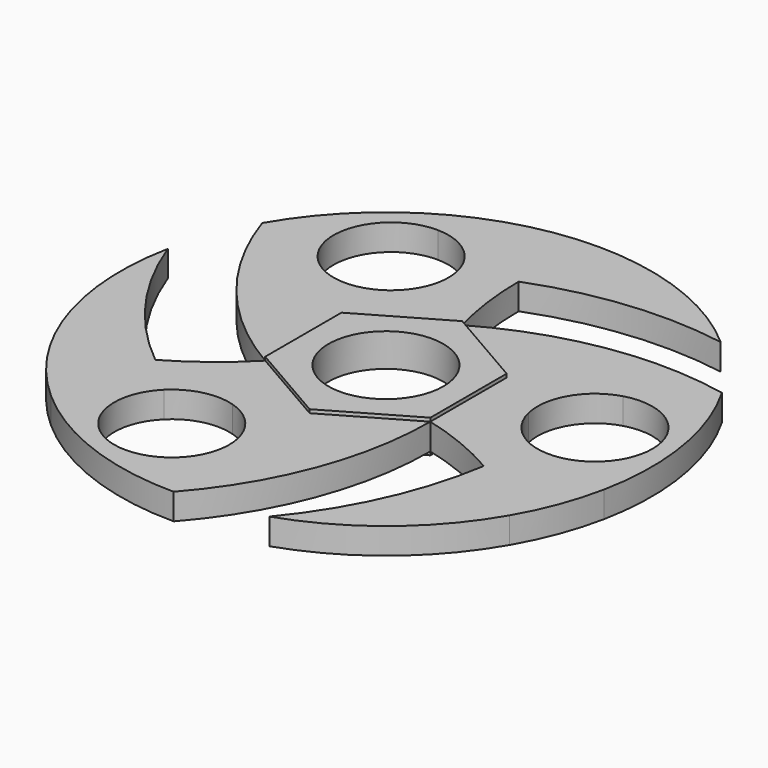
from build123d import *

# Parameters (mm, degrees)
F0_R     = 11
F1_DEPTH = 2.5
F2_DEPTH = 3.175


with BuildPart() as f1:
    # F0 (on Top) → F1 (new body, symmetric)
    with BuildSketch(Plane.XY):
        with BuildLine():
            ThreePointArc((20.292549, -3.190621), (15.603867, 0.493492), (10.5871, 3.716606))
            Line((10.5871, 3.716606), (10.5871, -14.535403))
            ThreePointArc((10.5871, -14.535403), (18.397515, -17.131664), (25.787001, -20.756393))
            ThreePointArc((25.787001, -20.756393), (32.620851, -25.343511), (38.774487, -30.809399))
            ThreePointArc((38.774487, -30.809399), (34.310981, -20.571216), (28.105483, -11.284932))
            ThreePointArc((28.105483, -11.284932), (23.085978, -8.312122), (20.292549, -3.190621))
        make_face()
        Polygon((10.5871, -14.535403), (10.5871, 3.716606), (-5.219603, 12.84261), (-21.026306, 3.716606), (-21.026306, -14.535403), (-5.219603, -23.661407), align=None)
        with Locations((-5.219603, -5.409399)):
            Circle(F0_R, mode=Mode.SUBTRACT)
        with BuildLine():
            Line((-5.219603, 12.84261), (10.5871, 3.716606))
            ThreePointArc((10.5871, 3.716606), (16.740736, 9.182493), (23.574586, 13.769612))
            ThreePointArc((23.574586, 13.769612), (30.964072, 17.39434), (38.774487, 19.990601))
            ThreePointArc((38.774487, 19.990601), (16.122412, 20.448153), (-5.219603, 12.84261))
        make_face()
        with BuildLine():
            ThreePointArc((-5.219603, -56.209399), (6.502686, -36.820901), (10.5871, -14.535403))
            Line((10.5871, -14.535403), (-5.219603, -23.661407))
            ThreePointArc((-5.219603, -23.661407), (-3.562824, -31.723556), (-3.007188, -39.935403))
            ThreePointArc((-3.007188, -39.935403), (-3.562824, -48.14725), (-5.219603, -56.209399))
        make_face()
        with BuildLine():
            Line((-21.026306, 3.716606), (-5.219603, 12.84261))
            ThreePointArc((-5.219603, 12.84261), (-6.876383, 20.904759), (-7.432019, 29.116606))
            ThreePointArc((-7.432019, 29.116606), (-6.876383, 37.328452), (-5.219603, 45.390601))
            ThreePointArc((-5.219603, 45.390601), (-11.854376, 36.406), (-16.793785, 26.388739))
            ThreePointArc((-16.793785, 26.388739), (-16.522621, 25.000927), (-16.431732, 23.589795))
            ThreePointArc((-16.431732, 23.589795), (-17.335201, 19.224012), (-19.897197, 15.575384))
            ThreePointArc((-19.897197, 15.575384), (-20.743392, 9.672811), (-21.026306, 3.716606))
        make_face()
        with BuildLine():
            ThreePointArc((38.774487, 19.990601), (30.964072, 17.39434), (23.574586, 13.769612))
            ThreePointArc((23.574586, 13.769612), (25.809021, 11.881337), (27.960245, 9.898783))
            ThreePointArc((27.960245, 9.898783), (37.61704, 8.114843), (42.0005, -0.672728))
            ThreePointArc((42.0005, -0.672728), (41.596743, -3.625628), (40.415115, -6.361755))
            ThreePointArc((40.415115, -6.361755), (42.663166, -10.833694), (44.576485, -15.458754))
            ThreePointArc((44.576485, -15.458754), (44.913356, 2.795866), (38.774487, 19.990601))
        make_face()
        with BuildLine():
            ThreePointArc((-16.054161, -28.612959), (-10.519285, -26.394499), (-5.219603, -23.661407))
            Line((-5.219603, -23.661407), (-21.026306, -14.535403))
            ThreePointArc((-21.026306, -14.535403), (-27.179942, -20.00129), (-34.013792, -24.588409))
            ThreePointArc((-34.013792, -24.588409), (-41.403278, -28.213137), (-49.213694, -30.809399))
            ThreePointArc((-49.213694, -30.809399), (-38.115414, -32.06298), (-26.970508, -31.332003))
            ThreePointArc((-26.970508, -31.332003), (-21.886226, -28.471389), (-16.054161, -28.612959))
        make_face()
        with BuildLine():
            ThreePointArc((38.774487, -30.809399), (32.620851, -25.343511), (25.787001, -20.756393))
            ThreePointArc((25.787001, -20.756393), (20.588854, -38.154406), (10.975444, -53.558754))
            ThreePointArc((10.975444, -53.558754), (26.952844, -44.723183), (38.774487, -30.809399))
        make_face()
        with BuildLine():
            ThreePointArc((-38.820645, -43.509399), (-23.180116, -52.928448), (-5.219603, -56.209399))
            ThreePointArc((-5.219603, -56.209399), (-3.562824, -48.14725), (-3.007188, -39.935403))
            ThreePointArc((-3.007188, -39.935403), (-5.759699, -40.926344), (-8.552253, -41.798082))
            ThreePointArc((-8.552253, -41.798082), (-17.801202, -50.052392), (-28.861727, -44.454046))
            ThreePointArc((-28.861727, -44.454046), (-33.858565, -44.164946), (-38.820645, -43.509399))
        make_face()
        with BuildLine():
            Line((-21.026306, -14.535403), (-21.026306, 3.716606))
            ThreePointArc((-21.026306, 3.716606), (-28.836722, 6.312867), (-36.226208, 9.937595))
            ThreePointArc((-36.226208, 9.937595), (-43.060058, 14.524714), (-49.213694, 19.990601))
            ThreePointArc((-49.213694, 19.990601), (-38.283907, 0.144553), (-21.026306, -14.535403))
        make_face()
        with BuildLine():
            ThreePointArc((-5.219603, 45.390601), (-6.876383, 37.328452), (-7.432019, 29.116606))
            ThreePointArc((-7.432019, 29.116606), (10.234176, 33.313884), (28.381438, 32.690601))
            ThreePointArc((28.381438, 32.690601), (12.740909, 42.10965), (-5.219603, 45.390601))
        make_face()
        with BuildLine():
            ThreePointArc((40.415115, -6.361755), (35.085314, -10.886165), (28.105483, -11.284932))
            ThreePointArc((28.105483, -11.284932), (34.310981, -20.571216), (38.774487, -30.809399))
            ThreePointArc((38.774487, -30.809399), (42.299445, -23.369911), (44.576485, -15.458754))
            ThreePointArc((44.576485, -15.458754), (42.663166, -10.833694), (40.415115, -6.361755))
        make_face()
        with BuildLine():
            ThreePointArc((-49.213694, -30.809399), (-44.533388, -37.581846), (-38.820645, -43.509399))
            ThreePointArc((-38.820645, -43.509399), (-33.858565, -44.164946), (-28.861727, -44.454046))
            ThreePointArc((-28.861727, -44.454046), (-30.115081, -37.576098), (-26.970508, -31.332003))
            ThreePointArc((-26.970508, -31.332003), (-38.115414, -32.06298), (-49.213694, -30.809399))
        make_face()
        with BuildLine():
            ThreePointArc((-49.213694, 19.990601), (-43.060058, 14.524714), (-36.226208, 9.937595))
            ThreePointArc((-36.226208, 9.937595), (-35.708132, 12.816811), (-35.066802, 15.671102))
            ThreePointArc((-35.066802, 15.671102), (-37.59077, 27.808082), (-27.212198, 34.587604))
            ThreePointArc((-27.212198, 34.587604), (-24.463411, 38.770444), (-21.41465, 42.739957))
            ThreePointArc((-21.41465, 42.739957), (-37.392051, 33.904386), (-49.213694, 19.990601))
        make_face()
        with BuildLine():
            ThreePointArc((-16.793785, 26.388739), (-11.854376, 36.406), (-5.219603, 45.390601))
            ThreePointArc((-5.219603, 45.390601), (-13.424868, 44.723561), (-21.41465, 42.739957))
            ThreePointArc((-21.41465, 42.739957), (-24.463411, 38.770444), (-27.212198, 34.587604))
            ThreePointArc((-27.212198, 34.587604), (-20.629043, 32.234067), (-16.793785, 26.388739))
        make_face()
        with BuildLine():
            ThreePointArc((-49.213694, -30.809399), (-41.403278, -28.213137), (-34.013792, -24.588409))
            ThreePointArc((-34.013792, -24.588409), (-46.48184, -11.387675), (-55.015692, 4.639957))
            ThreePointArc((-55.015692, 4.639957), (-55.352563, -13.614663), (-49.213694, -30.809399))
        make_face()
        with BuildLine():
            ThreePointArc((-36.226208, 9.937595), (-28.836722, 6.312867), (-21.026306, 3.716606))
            ThreePointArc((-21.026306, 3.716606), (-20.743392, 9.672811), (-19.897197, 15.575384))
            ThreePointArc((-19.897197, 15.575384), (-27.501139, 12.590014), (-35.066802, 15.671102))
            ThreePointArc((-35.066802, 15.671102), (-35.708132, 12.816811), (-36.226208, 9.937595))
        make_face()
        with BuildLine():
            ThreePointArc((23.574586, 13.769612), (16.740736, 9.182493), (10.5871, 3.716606))
            ThreePointArc((10.5871, 3.716606), (15.603867, 0.493492), (20.292549, -3.190621))
            ThreePointArc((20.292549, -3.190621), (21.509113, 4.887271), (27.960245, 9.898783))
            ThreePointArc((27.960245, 9.898783), (25.809021, 11.881337), (23.574586, 13.769612))
        make_face()
        with BuildLine():
            ThreePointArc((-3.007188, -39.935403), (-3.562824, -31.723556), (-5.219603, -23.661407))
            ThreePointArc((-5.219603, -23.661407), (-10.519285, -26.394499), (-16.054161, -28.612959))
            ThreePointArc((-16.054161, -28.612959), (-10.398433, -32.584302), (-8.227578, -39.145263))
            ThreePointArc((-8.227578, -39.145263), (-8.309048, -40.48157), (-8.552253, -41.798082))
            ThreePointArc((-8.552253, -41.798082), (-5.759699, -40.926344), (-3.007188, -39.935403))
        make_face()
    extrude(amount=F1_DEPTH, both=True)

    # F0 (on Top) → F2 (join, symmetric)
    with BuildSketch(Plane.XY):
        Polygon((10.5871, -14.535403), (10.5871, 3.716606), (-5.219603, 12.84261), (-21.026306, 3.716606), (-21.026306, -14.535403), (-5.219603, -23.661407), align=None)
        with Locations((-5.219603, -5.409399)):
            Circle(F0_R, mode=Mode.SUBTRACT)
    extrude(amount=F2_DEPTH, both=True)


solid = f1.part
